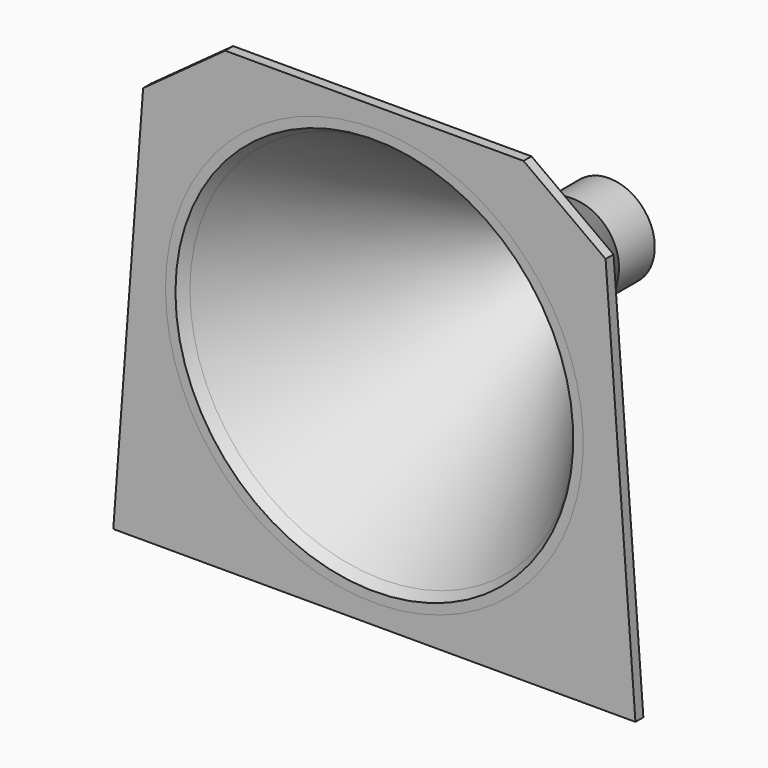
from build123d import *
from build123d import SkipClean  # not in build123d's __all__

# Parameters (mm, degrees)
F2_DEPTH = 2
F1_W     = 2
F1_H     = 9
F6_DEPTH = 3


with BuildPart() as f2:
    # F0 (on Front) → F2 (new body)
    with BuildSketch(Plane.XZ):
        Polygon((-52.5, -46), (52.5, -46), (46.5, 34), (30, 46), (-30, 46), (-46.5, 34), align=None)
    extrude(amount=-F2_DEPTH)

    # F1 (on Top) → F3 (revolve, cut)
    with BuildSketch(Plane.XY):
        Polygon((-20, 0), (0, 0), (0, 50), (-7.2, 50), (-40, 0), (-22, 0), align=None)
    revolve(axis=Axis((0, 25, 0), (0, 1, 0)), mode=Mode.SUBTRACT)

    # F1 (on Top) → F4 (revolve)
    with BuildSketch(Plane.XY):
        Polygon((-40, 0), (-7.2, 50), (-9.2, 50), (-42, 0), align=None)
        with Locations((-8.2, 54.5)):
            Rectangle(F1_W, F1_H)
    with SkipClean():  # cleaning this boolean's faces spoils the solid; the shape is the same uncleaned
        revolve(axis=Axis((0, 2, 0), (0, -1, 0)))

    # F5 (on face) → F6 (join)
    with BuildSketch(Plane(origin=(0, 59, 0), x_dir=(-1, 0, 0), z_dir=(0, 1, 0))):
        with BuildLine():
            Line((-6.2, -3.6606010435), (-6.2, 0))
            Line((-6.2, 0), (-6.2, 3.6606010435))
            ThreePointArc((-6.2, 3.6606010435), (-7.2, 0), (-6.2, -3.6606010435))
        make_face()
        with BuildLine():
            ThreePointArc((7.2, 0), (6.9455021417, 1.8973665961), (6.2, 3.6606010435))
            Line((6.2, 3.6606010435), (6.2, -3.6606010435))
            ThreePointArc((6.2, -3.6606010435), (6.9455021417, -1.8973665961), (7.2, 0))
        make_face()
    with SkipClean():  # cleaning this boolean's faces spoils the solid; the shape is the same uncleaned
        extrude(amount=-F6_DEPTH)


solid = f2.part
